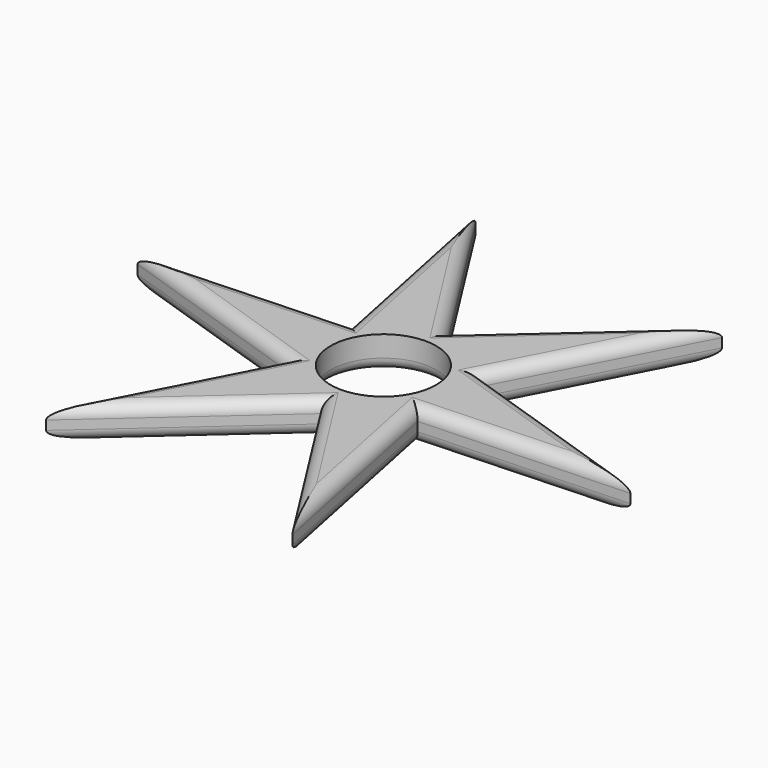
from build123d import *

# Parameters (mm, degrees)
F0_R          = 11.2395
F1_DEPTH      = 7.0104
F2_R          = 2.54
F3_T4_DEPTH   = 58.4517099093
F3_T9_DEPTH   = 56.5105690907
F3_T14_DEPTH  = 58.4517099093
F3_T19_DEPTH  = 56.5105690907
F3_T24_DEPTH  = 58.4517099093
F3_T29_DEPTH  = 56.5105690907
F3_T34_DEPTH  = 58.4517099093
F3_T39_DEPTH  = 56.5105690907
F3_T44_DEPTH  = 58.4517099093
F3_T49_DEPTH  = 56.5105690907
F3_T54_DEPTH  = 58.4517099093
F3_T59_DEPTH  = 56.5105690907
F3_T67_DEPTH  = 58.4517099093
F3_T71_DEPTH  = 56.5105690907
F3_T78_DEPTH  = 58.4517099093
F3_T82_DEPTH  = 56.5105690907
F3_T89_DEPTH  = 58.4517099093
F3_T93_DEPTH  = 56.5105690907
F3_T100_DEPTH = 58.4517099093
F3_T104_DEPTH = 56.5105690907
F3_T111_DEPTH = 58.4517099093
F3_T115_DEPTH = 56.5105690907
F3_T122_DEPTH = 56.5105690907
F3_T126_DEPTH = 58.4517099093


# Not quite as in the source:
# - a fillet or chamfer that OpenCascade refuses, or shapes differently, is made with other operations: its cross-section is extruded or revolved along the edge and cut away or added


with BuildPart() as f1:
    # F0 (on Top) → F1 (new body)
    with BuildSketch(Plane.XY):
        with BuildLine():
            ThreePointArc((14.1535943712, 7.539855096), (15.5587542777, 3.8857192152), (16.036634575, 0))
            ThreePointArc((16.036634575, 0), (15.49765005, -4.122680126), (13.91692656, -7.9682371712))
            Line((13.91692656, -7.9682371712), (13.9999523741, -8.373134936))
            Line((13.9999523741, -8.373134936), (57.7710043319, -6.5127654675))
            Line((57.7710043319, -6.5127654675), (14.3613089772, 7.9377469398))
            Line((14.3613089772, 7.9377469398), (14.1535943712, 7.539855096))
        make_face()
        with BuildLine():
            ThreePointArc((0, 16.036634575), (8.2540822497, 13.7493190635), (14.1535943712, 7.539855096))
            Line((14.1535943712, 7.539855096), (14.3613089772, 7.9377469398))
            Line((14.3613089772, 7.9377469398), (34.635707736, 46.7747746198))
            Line((34.635707736, 46.7747746198), (0.4163492162, 16.4061318757))
            Line((0.4163492162, 16.4061318757), (0, 16.036634575))
        make_face()
        with BuildLine():
            Line((13.9999523741, -8.373134936), (13.91692656, -7.9682371712))
            ThreePointArc((13.91692656, -7.9682371712), (13.7943089537, -8.1786728131), (13.6685096291, -8.387222008))
            Line((13.6685096291, -8.387222008), (13.9999523741, -8.373134936))
        make_face()
        with BuildLine():
            ThreePointArc((-13.549530457, 8.5781042712), (-7.7333603611, 14.048800163), (0, 16.036634575))
            Line((0, 16.036634575), (0.4163492162, 16.4061318757))
            Line((0.4163492162, 16.4061318757), (-23.0803039828, 53.3827900874))
            Line((-23.0803039828, 53.3827900874), (-13.8899671478, 8.563634936))
            Line((-13.8899671478, 8.563634936), (-13.549530457, 8.5781042712))
        make_face()
        with BuildLine():
            Line((13.9999523741, -8.373134936), (13.6685096291, -8.387222008))
            ThreePointArc((13.6685096291, -8.387222008), (7.7861485351, -14.0196126723), (-0.1042878985, -16.036295474))
            Line((-0.1042878985, -16.036295474), (-0.30636399, -16.2156318757))
            Line((-0.30636399, -16.2156318757), (23.190289209, -53.1922900874))
            Line((23.190289209, -53.1922900874), (13.9999523741, -8.373134936))
        make_face()
        with BuildLine():
            ThreePointArc((-13.8067270062, 8.157691945), (-13.6797438656, 8.3688862021), (-13.549530457, 8.5781042712))
            Line((-13.549530457, 8.5781042712), (-13.8899671478, 8.563634936))
            Line((-13.8899671478, 8.563634936), (-13.8067270062, 8.157691945))
        make_face()
        with BuildLine():
            Line((-0.30636399, -16.2156318757), (-0.1042878985, -16.036295474))
            ThreePointArc((-0.1042878985, -16.036295474), (-0.2639889319, -16.0344615855), (-0.4236637816, -16.0310373181))
            Line((-0.4236637816, -16.0310373181), (-0.30636399, -16.2156318757))
        make_face()
        with BuildLine():
            ThreePointArc((-14.1482702845, -7.5498408229), (-16.0328448753, 0.3486168375), (-13.8067270062, 8.157691945))
            Line((-13.8067270062, 8.157691945), (-13.8899671478, 8.563634936))
            Line((-13.8899671478, 8.563634936), (-57.6610191056, 6.7032654675))
            Line((-57.6610191056, 6.7032654675), (-14.2513237509, -7.7472469398))
            Line((-14.2513237509, -7.7472469398), (-14.1482702845, -7.5498408229))
        make_face()
        with BuildLine():
            Line((-0.30636399, -16.2156318757), (-0.4236637816, -16.0310373181))
            ThreePointArc((-0.4236637816, -16.0310373181), (-8.2924525996, -13.7262113628), (-13.9934373276, -7.8330939131))
            Line((-13.9934373276, -7.8330939131), (-14.2513237509, -7.7472469398))
            Line((-14.2513237509, -7.7472469398), (-34.5257225097, -46.5842746198))
            Line((-34.5257225097, -46.5842746198), (-0.30636399, -16.2156318757))
        make_face()
        with BuildLine():
            ThreePointArc((-13.9934373276, -7.8330939131), (-14.0715665407, -7.6918569659), (-14.1482702845, -7.5498408229))
            Line((-14.1482702845, -7.5498408229), (-14.2513237509, -7.7472469398))
            Line((-14.2513237509, -7.7472469398), (-13.9934373276, -7.8330939131))
        make_face()
        with BuildLine():
            ThreePointArc((13.91692656, -7.9682371712), (15.49765005, -4.122680126), (16.036634575, 0))
            ThreePointArc((16.036634575, 0), (15.5587542777, 3.8857192152), (14.1535943712, 7.539855096))
            ThreePointArc((14.1535943712, 7.539855096), (8.2540822497, 13.7493190635), (0, 16.036634575))
            ThreePointArc((0, 16.036634575), (-7.7333603611, 14.048800163), (-13.549530457, 8.5781042712))
            ThreePointArc((-13.549530457, 8.5781042712), (-13.6797438656, 8.3688862021), (-13.8067270062, 8.157691945))
            ThreePointArc((-13.8067270062, 8.157691945), (-16.0328448753, 0.3486168375), (-14.1482702845, -7.5498408229))
            ThreePointArc((-14.1482702845, -7.5498408229), (-14.0715665407, -7.6918569659), (-13.9934373276, -7.8330939131))
            ThreePointArc((-13.9934373276, -7.8330939131), (-8.2924525996, -13.7262113628), (-0.4236637816, -16.0310373181))
            ThreePointArc((-0.4236637816, -16.0310373181), (-0.2639889319, -16.0344615855), (-0.1042878985, -16.036295474))
            ThreePointArc((-0.1042878985, -16.036295474), (7.7861485351, -14.0196126723), (13.6685096291, -8.387222008))
            ThreePointArc((13.6685096291, -8.387222008), (13.7943089537, -8.1786728131), (13.91692656, -7.9682371712))
        make_face()
        Circle(F0_R, mode=Mode.SUBTRACT)
    extrude(amount=F1_DEPTH)

    # F2
    f2_edges = [f1.edges().sort_by_distance(p)[0] for p in [
        (36.066157, 0.712491, 7.0104),
        (24.498508, 27.356261, 7.0104),
        (17.526028, 31.590453, 7.0104),
        (-11.331977, 34.894461, 7.0104),
        (-18.485136, 30.973213, 7.0104),
        (-35.775493, 7.63345, 7.0104),
        (-35.956171, -0.521991, 7.0104),
        (-24.388523, -27.165761, 7.0104),
        (-17.416043, -31.399953, 7.0104),
        (11.441963, -34.703961, 7.0104),
        (18.595121, -30.782713, 7.0104),
        (35.885478, -7.44295, 7.0104),
    ]]
    fillet(f2_edges, radius=F2_R)

    # F3: fillet of radius 2.54 on 13 edges, made by hand


with BuildPart() as f3_tool2:
    # F3_s3 → F3_t4 (new body)
    with BuildSketch(Plane(origin=(-59.9425858258, 19.9540925852, 0), x_dir=(0, 0, 1), z_dir=(0.9488103383, -0.3158463899, 0))):
        with BuildLine():
            ThreePointArc((2.54, 11.8518971477), (0.7439487758, 11.1079483719), (0, 9.3118971477))
            Line((0, 9.3118971477), (0, 11.8518971477))
            Line((0, 11.8518971477), (2.54, 11.8518971477))
        make_face()
    extrude(amount=F3_T4_DEPTH)

    split(bisect_by=Plane(origin=(-8.0210442823, 4.1872887797, 0), x_dir=(0, 0, 1), z_dir=(-0.8864762199, 0.4627741474, 0)), keep=Keep.TOP)


with BuildPart() as f1_1:
    add(f1.part)

    # F3_t1: cut F3_tool2
    add(f3_tool2.part, mode=Mode.SUBTRACT)


with BuildPart() as f3_tool7:
    # F3_s8 → F3_t9 (new body)
    with BuildSketch(Plane(origin=(-3.2916636325, -6.305411723, 0), x_dir=(0, 0, 1), z_dir=(-0.4627741474, -0.8864762199, 0))):
        with BuildLine():
            ThreePointArc((0, 6.5082340102), (0.7439487758, 8.3042852344), (2.54, 9.0482340102))
            Line((2.54, 9.0482340102), (0, 9.0482340102))
            Line((0, 9.0482340102), (0, 6.5082340102))
        make_face()
    extrude(amount=F3_T9_DEPTH)

    split(bisect_by=Plane(origin=(-3.7433789278, -11.2452025417, 0), x_dir=(0, 0, 1), z_dir=(-0.3158463899, -0.9488103383, 0)), keep=Keep.TOP)


with BuildPart() as f1_2:
    add(f1_1.part)

    # F3_t6: cut F3_tool7
    add(f3_tool7.part, mode=Mode.SUBTRACT)


with BuildPart() as f3_tool12:
    # F3_s13 → F3_t14 (new body)
    with BuildSketch(Plane(origin=(-47.1905173297, -41.8801527464, 0), x_dir=(0, 0, 1), z_dir=(0.7479361665, 0.6637706613, 0))):
        with BuildLine():
            ThreePointArc((0, 9.3849021141), (0.7439487758, 11.1809533383), (2.54, 11.9249021141))
            Line((2.54, 11.9249021141), (0, 11.9249021141))
            Line((0, 11.9249021141), (0, 9.3849021141))
        make_face()
    extrude(amount=F3_T14_DEPTH)

    split(bisect_by=Plane(origin=(-7.5584718817, -4.8029973802, 0), x_dir=(0, 0, 1), z_dir=(-0.8440122778, -0.5363238526, 0)), keep=Keep.TOP)


with BuildPart() as f1_3:
    add(f1_2.part)

    # F3_t11: cut F3_tool12
    add(f3_tool12.part, mode=Mode.SUBTRACT)


with BuildPart() as f3_tool17:
    # F3_s18 → F3_t19 (new body)
    with BuildSketch(Plane(origin=(3.8464514278, -6.0531565313, 0), x_dir=(0, 0, 1), z_dir=(0.5363238526, -0.8440122778, 0))):
        with BuildLine():
            ThreePointArc((0, 6.4154051288), (0.7439487758, 8.211456353), (2.54, 8.9554051288))
            Line((2.54, 8.9554051288), (0, 8.9554051288))
            Line((0, 8.9554051288), (0, 6.4154051288))
        make_face()
    extrude(amount=F3_T19_DEPTH)

    split(bisect_by=Plane(origin=(7.9154001627, -8.9190655729, 0), x_dir=(0, 0, 1), z_dir=(0.6637706613, -0.7479361665, 0)), keep=Keep.TOP)


with BuildPart() as f1_4:
    add(f1_3.part)

    # F3_t16: cut F3_tool17
    add(f3_tool17.part, mode=Mode.SUBTRACT)


with BuildPart() as f3_tool22:
    # F3_s23 → F3_t24 (new body)
    with BuildSketch(Plane(origin=(12.6784554794, -61.8299060653, 0), x_dir=(0, 0, 1), z_dir=(-0.2008741718, 0.9796170513, 0))):
        with BuildLine():
            ThreePointArc((0, 9.4926455171), (0.7439487758, 11.2886967414), (2.54, 12.0326455171))
            Line((2.54, 12.0326455171), (0, 12.0326455171))
            Line((0, 12.0326455171), (0, 9.4926455171))
        make_face()
    extrude(amount=F3_T24_DEPTH)

    split(bisect_by=Plane(origin=(0.3804801286, -8.9519935471, 0), x_dir=(0, 0, 1), z_dir=(0.0424639421, -0.999098, 0)), keep=Keep.TOP)


with BuildPart() as f1_5:
    add(f1_4.part)

    # F3_t21: cut F3_tool22
    add(f3_tool22.part, mode=Mode.SUBTRACT)


with BuildPart() as f3_tool27:
    # F3_s28 → F3_t29 (new body)
    with BuildSketch(Plane(origin=(7.2751999455, 0.3092125789, 0), x_dir=(0, 0, 1), z_dir=(0.999098, 0.0424639421, 0))):
        with BuildLine():
            ThreePointArc((0, 6.4200755351), (0.7439487758, 8.2161267593), (2.54, 8.9600755351))
            Line((2.54, 8.9600755351), (0, 8.9600755351))
            Line((0, 8.9600755351), (0, 6.4200755351))
        make_face()
    extrude(amount=F3_T29_DEPTH)

    split(bisect_by=Plane(origin=(11.7873847203, 2.4170477024, 0), x_dir=(0, 0, 1), z_dir=(0.9796170513, 0.2008741718, 0)), keep=Keep.TOP)


with BuildPart() as f1_6:
    add(f1_5.part)

    # F3_t26: cut F3_tool27
    add(f3_tool27.part, mode=Mode.SUBTRACT)


with BuildPart() as f3_tool32:
    # F3_s33 → F3_t34 (new body)
    with BuildSketch(Plane(origin=(59.9845103223, -19.9680486945, 0), x_dir=(0, 0, 1), z_dir=(-0.9488103383, 0.3158463899, 0))):
        with BuildLine():
            ThreePointArc((0, 9.5273839538), (0.7439487758, 11.323435178), (2.54, 12.0673839538))
            Line((2.54, 12.0673839538), (0, 12.0673839538))
            Line((0, 12.0673839538), (0, 9.5273839538))
        make_face()
    extrude(amount=F3_T34_DEPTH)

    split(bisect_by=Plane(origin=(8.0293246905, -4.1916114663, 0), x_dir=(0, 0, 1), z_dir=(0.8864762199, -0.4627741474, 0)), keep=Keep.TOP)


with BuildPart() as f1_7:
    add(f1_6.part)

    # F3_t31: cut F3_tool32
    add(f3_tool32.part, mode=Mode.SUBTRACT)


with BuildPart() as f3_tool37:
    # F3_s38 → F3_t39 (new body)
    with BuildSketch(Plane(origin=(3.3933684506, 6.5002344095, 0), x_dir=(0, 0, 1), z_dir=(0.4627741474, 0.8864762199, 0))):
        with BuildLine():
            ThreePointArc((0, 6.5175748228), (0.7439487758, 8.313626047), (2.54, 9.0575748228))
            Line((2.54, 9.0575748228), (0, 9.0575748228))
            Line((0, 9.0575748228), (0, 6.5175748228))
        make_face()
    extrude(amount=F3_T39_DEPTH)

    split(bisect_by=Plane(origin=(3.8114396575, 11.449658651, 0), x_dir=(0, 0, 1), z_dir=(0.3158463899, 0.9488103383, 0)), keep=Keep.TOP)


with BuildPart() as f1_8:
    add(f1_7.part)

    # F3_t36: cut F3_tool37
    add(f3_tool37.part, mode=Mode.SUBTRACT)


with BuildPart() as f3_tool42:
    # F3_s43 → F3_t44 (new body)
    with BuildSketch(Plane(origin=(47.3466192661, 42.0186884801, 0), x_dir=(0, 0, 1), z_dir=(-0.7479361665, -0.6637706613, 0))):
        with BuildLine():
            ThreePointArc((0, 9.4543789874), (0.7439487758, 11.2504302116), (2.54, 11.9943789874))
            Line((2.54, 11.9943789874), (0, 11.9943789874))
            Line((0, 11.9943789874), (0, 9.4543789874))
        make_face()
    extrude(amount=F3_T44_DEPTH)

    split(bisect_by=Plane(origin=(7.7230530734, 4.9075797674, 0), x_dir=(0, 0, 1), z_dir=(0.8440122778, 0.5363238526, 0)), keep=Keep.TOP)


with BuildPart() as f1_9:
    add(f1_8.part)

    # F3_t41: cut F3_tool42
    add(f3_tool42.part, mode=Mode.SUBTRACT)


with BuildPart() as f3_tool47:
    # F3_s48 → F3_t49 (new body)
    with BuildSketch(Plane(origin=(-3.9010473932, 6.1390741441, 0), x_dir=(0, 0, 1), z_dir=(-0.5363238526, 0.8440122778, 0))):
        with BuildLine():
            ThreePointArc((0, 6.6104037041), (0.7439487758, 8.4064549283), (2.54, 9.1504037041))
            Line((2.54, 9.1504037041), (0, 9.1504037041))
            Line((0, 9.1504037041), (0, 6.6104037041))
        make_face()
    extrude(amount=F3_T49_DEPTH)

    split(bisect_by=Plane(origin=(-7.9615168729, 8.9710298392, 0), x_dir=(0, 0, 1), z_dir=(-0.6637706613, 0.7479361665, 0)), keep=Keep.TOP)


with BuildPart() as f1_10:
    add(f1_9.part)

    # F3_t46: cut F3_tool47
    add(f3_tool47.part, mode=Mode.SUBTRACT)


with BuildPart() as f3_tool52:
    # F3_s53 → F3_t54 (new body)
    with BuildSketch(Plane(origin=(-12.7115040729, 61.9910764409, 0), x_dir=(0, 0, 1), z_dir=(0.2008741718, -0.9796170513, 0))):
        with BuildLine():
            ThreePointArc((0, 9.3466355844), (0.7439487758, 11.1426868086), (2.54, 11.8866355844))
            Line((2.54, 11.8866355844), (0, 11.8866355844))
            Line((0, 11.8866355844), (0, 9.3466355844))
        make_face()
    extrude(amount=F3_T54_DEPTH)

    split(bisect_by=Plane(origin=(-0.3883638891, 9.1374838465, 0), x_dir=(0, 0, 1), z_dir=(-0.0424639421, 0.999098, 0)), keep=Keep.TOP)


with BuildPart() as f1_11:
    add(f1_10.part)

    # F3_t51: cut F3_tool52
    add(f3_tool52.part, mode=Mode.SUBTRACT)


with BuildPart() as f3_tool57:
    # F3_s58 → F3_t59 (new body)
    with BuildSketch(Plane(origin=(-7.1573309587, -0.3042028783, 0), x_dir=(0, 0, 1), z_dir=(-0.999098, -0.0424639421, 0))):
        with BuildLine():
            ThreePointArc((2.54, 9.1457332978), (0.7439487758, 8.4017845221), (0, 6.6057332978))
            Line((0, 6.6057332978), (0, 9.1457332978))
            Line((0, 9.1457332978), (2.54, 9.1457332978))
        make_face()
    extrude(amount=F3_T59_DEPTH)

    split(bisect_by=Plane(origin=(-11.6443509005, -2.3877180781, 0), x_dir=(0, 0, 1), z_dir=(-0.9796170513, -0.2008741718, 0)), keep=Keep.TOP)


with BuildPart() as f1_12:
    add(f1_11.part)

    # F3_t56: cut F3_tool57
    add(f3_tool57.part, mode=Mode.SUBTRACT)

    # F3_s61 → F3_t62 (revolve, cut)
    with BuildSketch(Plane.XZ):
        with BuildLine():
            ThreePointArc((13.7795, 0), (11.9834487758, 0.7439487758), (11.2395, 2.54))
            Line((11.2395, 2.54), (11.2395, 0))
            Line((11.2395, 0), (13.7795, 0))
        make_face()
    revolve(axis=Axis((0, 0, 0), (0, 0, 1)), mode=Mode.SUBTRACT)


with BuildPart() as f3_tool65:
    # F3_s66 → F3_t67 (new body)
    with BuildSketch(Plane(origin=(-59.9425858258, 19.9540925852, 0), x_dir=(0, 0, 1), z_dir=(0.9488103383, -0.3158463899, 0))):
        with BuildLine():
            ThreePointArc((2.54, 11.8518971477), (0.7439487758, 11.1079483719), (0, 9.3118971477))
            Line((0, 9.3118971477), (0, 11.8518971477))
            Line((0, 11.8518971477), (2.54, 11.8518971477))
        make_face()
    extrude(amount=F3_T67_DEPTH)

    split(bisect_by=Plane(origin=(-8.0210442823, 4.1872887797, 0), x_dir=(0, 0, 1), z_dir=(0.8864762199, -0.4627741474, 0)), keep=Keep.TOP)


with BuildPart() as f3_tool69:
    # F3_s70 → F3_t71 (new body)
    with BuildSketch(Plane(origin=(-3.2916636325, -6.305411723, 0), x_dir=(0, 0, 1), z_dir=(-0.4627741474, -0.8864762199, 0))):
        with BuildLine():
            ThreePointArc((0, 6.5082340102), (0.7439487758, 8.3042852344), (2.54, 9.0482340102))
            Line((2.54, 9.0482340102), (0, 9.0482340102))
            Line((0, 9.0482340102), (0, 6.5082340102))
        make_face()
    extrude(amount=F3_T71_DEPTH)

    split(bisect_by=Plane(origin=(-3.7433789278, -11.2452025417, 0), x_dir=(0, 0, 1), z_dir=(0.3158463899, 0.9488103383, 0)), keep=Keep.TOP)


with BuildPart() as f3_tool65_1:
    add(f3_tool65.part)

    # F3_t73: intersect F3_tool69
    add(f3_tool69.part, mode=Mode.INTERSECT)


with BuildPart() as f1_13:
    add(f1_12.part)

    # F3_t63: cut F3_tool65
    add(f3_tool65_1.part, mode=Mode.SUBTRACT)


with BuildPart() as f3_tool76:
    # F3_s77 → F3_t78 (new body)
    with BuildSketch(Plane(origin=(-47.1905173297, -41.8801527464, 0), x_dir=(0, 0, 1), z_dir=(0.7479361665, 0.6637706613, 0))):
        with BuildLine():
            ThreePointArc((0, 9.3849021141), (0.7439487758, 11.1809533383), (2.54, 11.9249021141))
            Line((2.54, 11.9249021141), (0, 11.9249021141))
            Line((0, 11.9249021141), (0, 9.3849021141))
        make_face()
    extrude(amount=F3_T78_DEPTH)

    split(bisect_by=Plane(origin=(-7.5584718817, -4.8029973802, 0), x_dir=(0, 0, 1), z_dir=(0.8440122778, 0.5363238526, 0)), keep=Keep.TOP)


with BuildPart() as f3_tool80:
    # F3_s81 → F3_t82 (new body)
    with BuildSketch(Plane(origin=(3.8464514278, -6.0531565313, 0), x_dir=(0, 0, 1), z_dir=(0.5363238526, -0.8440122778, 0))):
        with BuildLine():
            ThreePointArc((0, 6.4154051288), (0.7439487758, 8.211456353), (2.54, 8.9554051288))
            Line((2.54, 8.9554051288), (0, 8.9554051288))
            Line((0, 8.9554051288), (0, 6.4154051288))
        make_face()
    extrude(amount=F3_T82_DEPTH)

    split(bisect_by=Plane(origin=(7.9154001627, -8.9190655729, 0), x_dir=(0, 0, 1), z_dir=(-0.6637706613, 0.7479361665, 0)), keep=Keep.TOP)


with BuildPart() as f3_tool76_1:
    add(f3_tool76.part)

    # F3_t84: intersect F3_tool80
    add(f3_tool80.part, mode=Mode.INTERSECT)


with BuildPart() as f1_14:
    add(f1_13.part)

    # F3_t74: cut F3_tool76
    add(f3_tool76_1.part, mode=Mode.SUBTRACT)


with BuildPart() as f3_tool87:
    # F3_s88 → F3_t89 (new body)
    with BuildSketch(Plane(origin=(12.6784554794, -61.8299060653, 0), x_dir=(0, 0, 1), z_dir=(-0.2008741718, 0.9796170513, 0))):
        with BuildLine():
            ThreePointArc((0, 9.4926455171), (0.7439487758, 11.2886967414), (2.54, 12.0326455171))
            Line((2.54, 12.0326455171), (0, 12.0326455171))
            Line((0, 12.0326455171), (0, 9.4926455171))
        make_face()
    extrude(amount=F3_T89_DEPTH)

    split(bisect_by=Plane(origin=(0.3804801286, -8.9519935471, 0), x_dir=(0, 0, 1), z_dir=(-0.0424639421, 0.999098, 0)), keep=Keep.TOP)


with BuildPart() as f3_tool91:
    # F3_s92 → F3_t93 (new body)
    with BuildSketch(Plane(origin=(7.2751999455, 0.3092125789, 0), x_dir=(0, 0, 1), z_dir=(0.999098, 0.0424639421, 0))):
        with BuildLine():
            ThreePointArc((0, 6.4200755351), (0.7439487758, 8.2161267593), (2.54, 8.9600755351))
            Line((2.54, 8.9600755351), (0, 8.9600755351))
            Line((0, 8.9600755351), (0, 6.4200755351))
        make_face()
    extrude(amount=F3_T93_DEPTH)

    split(bisect_by=Plane(origin=(11.7873847203, 2.4170477024, 0), x_dir=(0, 0, 1), z_dir=(-0.9796170513, -0.2008741718, 0)), keep=Keep.TOP)


with BuildPart() as f3_tool87_1:
    add(f3_tool87.part)

    # F3_t95: intersect F3_tool91
    add(f3_tool91.part, mode=Mode.INTERSECT)


with BuildPart() as f1_15:
    add(f1_14.part)

    # F3_t85: cut F3_tool87
    add(f3_tool87_1.part, mode=Mode.SUBTRACT)


with BuildPart() as f3_tool98:
    # F3_s99 → F3_t100 (new body)
    with BuildSketch(Plane(origin=(59.9845103223, -19.9680486945, 0), x_dir=(0, 0, 1), z_dir=(-0.9488103383, 0.3158463899, 0))):
        with BuildLine():
            ThreePointArc((0, 9.5273839538), (0.7439487758, 11.323435178), (2.54, 12.0673839538))
            Line((2.54, 12.0673839538), (0, 12.0673839538))
            Line((0, 12.0673839538), (0, 9.5273839538))
        make_face()
    extrude(amount=F3_T100_DEPTH)

    split(bisect_by=Plane(origin=(8.0293246905, -4.1916114663, 0), x_dir=(0, 0, 1), z_dir=(-0.8864762199, 0.4627741474, 0)), keep=Keep.TOP)


with BuildPart() as f3_tool102:
    # F3_s103 → F3_t104 (new body)
    with BuildSketch(Plane(origin=(3.3933684506, 6.5002344095, 0), x_dir=(0, 0, 1), z_dir=(0.4627741474, 0.8864762199, 0))):
        with BuildLine():
            ThreePointArc((0, 6.5175748228), (0.7439487758, 8.313626047), (2.54, 9.0575748228))
            Line((2.54, 9.0575748228), (0, 9.0575748228))
            Line((0, 9.0575748228), (0, 6.5175748228))
        make_face()
    extrude(amount=F3_T104_DEPTH)

    split(bisect_by=Plane(origin=(3.8114396575, 11.449658651, 0), x_dir=(0, 0, 1), z_dir=(-0.3158463899, -0.9488103383, 0)), keep=Keep.TOP)


with BuildPart() as f3_tool98_1:
    add(f3_tool98.part)

    # F3_t106: intersect F3_tool102
    add(f3_tool102.part, mode=Mode.INTERSECT)


with BuildPart() as f1_16:
    add(f1_15.part)

    # F3_t96: cut F3_tool98
    add(f3_tool98_1.part, mode=Mode.SUBTRACT)


with BuildPart() as f3_tool109:
    # F3_s110 → F3_t111 (new body)
    with BuildSketch(Plane(origin=(47.3466192661, 42.0186884801, 0), x_dir=(0, 0, 1), z_dir=(-0.7479361665, -0.6637706613, 0))):
        with BuildLine():
            ThreePointArc((0, 9.4543789874), (0.7439487758, 11.2504302116), (2.54, 11.9943789874))
            Line((2.54, 11.9943789874), (0, 11.9943789874))
            Line((0, 11.9943789874), (0, 9.4543789874))
        make_face()
    extrude(amount=F3_T111_DEPTH)

    split(bisect_by=Plane(origin=(7.7230530734, 4.9075797674, 0), x_dir=(0, 0, 1), z_dir=(-0.8440122778, -0.5363238526, 0)), keep=Keep.TOP)


with BuildPart() as f3_tool113:
    # F3_s114 → F3_t115 (new body)
    with BuildSketch(Plane(origin=(-3.9010473932, 6.1390741441, 0), x_dir=(0, 0, 1), z_dir=(-0.5363238526, 0.8440122778, 0))):
        with BuildLine():
            ThreePointArc((0, 6.6104037041), (0.7439487758, 8.4064549283), (2.54, 9.1504037041))
            Line((2.54, 9.1504037041), (0, 9.1504037041))
            Line((0, 9.1504037041), (0, 6.6104037041))
        make_face()
    extrude(amount=F3_T115_DEPTH)

    split(bisect_by=Plane(origin=(-7.9615168729, 8.9710298392, 0), x_dir=(0, 0, 1), z_dir=(0.6637706613, -0.7479361665, 0)), keep=Keep.TOP)


with BuildPart() as f3_tool109_1:
    add(f3_tool109.part)

    # F3_t117: intersect F3_tool113
    add(f3_tool113.part, mode=Mode.INTERSECT)


with BuildPart() as f1_17:
    add(f1_16.part)

    # F3_t107: cut F3_tool109
    add(f3_tool109_1.part, mode=Mode.SUBTRACT)


with BuildPart() as f3_tool120:
    # F3_s121 → F3_t122 (new body)
    with BuildSketch(Plane(origin=(-7.1573309587, -0.3042028783, 0), x_dir=(0, 0, 1), z_dir=(-0.999098, -0.0424639421, 0))):
        with BuildLine():
            ThreePointArc((2.54, 9.1457332978), (0.7439487758, 8.4017845221), (0, 6.6057332978))
            Line((0, 6.6057332978), (0, 9.1457332978))
            Line((0, 9.1457332978), (2.54, 9.1457332978))
        make_face()
    extrude(amount=F3_T122_DEPTH)

    split(bisect_by=Plane(origin=(-11.6443509005, -2.3877180781, 0), x_dir=(0, 0, 1), z_dir=(0.9796170513, 0.2008741718, 0)), keep=Keep.TOP)


with BuildPart() as f3_tool124:
    # F3_s125 → F3_t126 (new body)
    with BuildSketch(Plane(origin=(-12.7115040729, 61.9910764409, 0), x_dir=(0, 0, 1), z_dir=(0.2008741718, -0.9796170513, 0))):
        with BuildLine():
            ThreePointArc((0, 9.3466355844), (0.7439487758, 11.1426868086), (2.54, 11.8866355844))
            Line((2.54, 11.8866355844), (0, 11.8866355844))
            Line((0, 11.8866355844), (0, 9.3466355844))
        make_face()
    extrude(amount=F3_T126_DEPTH)

    split(bisect_by=Plane(origin=(-0.3883638891, 9.1374838465, 0), x_dir=(0, 0, 1), z_dir=(0.0424639421, -0.999098, 0)), keep=Keep.TOP)


with BuildPart() as f3_tool120_1:
    add(f3_tool120.part)

    # F3_t128: intersect F3_tool124
    add(f3_tool124.part, mode=Mode.INTERSECT)


with BuildPart() as f1_18:
    add(f1_17.part)

    # F3_t118: cut F3_tool120
    add(f3_tool120_1.part, mode=Mode.SUBTRACT)


solid = f1_18.part
